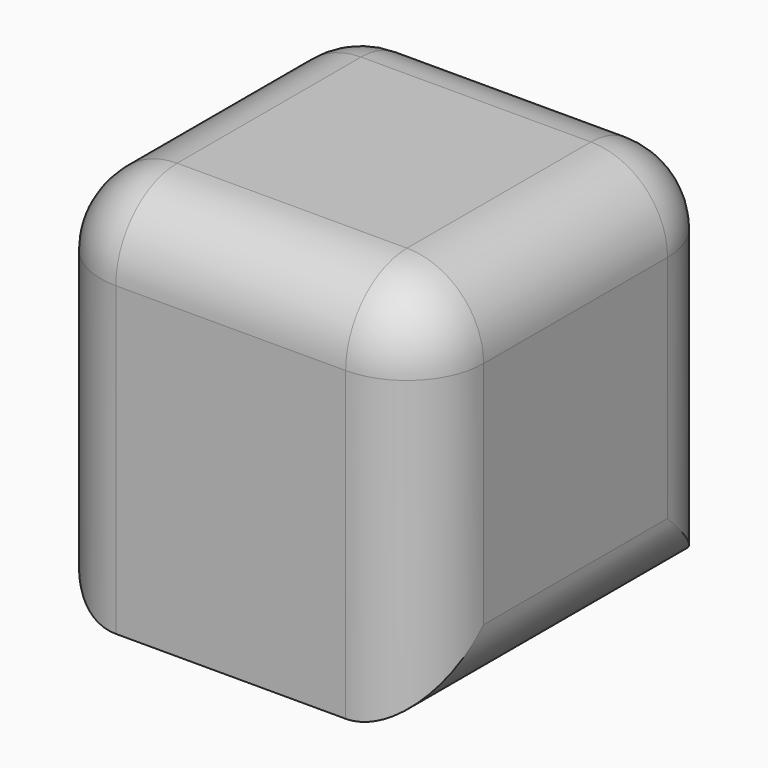
from build123d import *

# Parameters (mm, degrees)
F0_W         = 25
F0_H         = 25
F1_DEPTH     = 25
F2_T         = -3
F3_T1_DEPTH  = 32.5
F3_T3_DEPTH  = 50
F3_T5_DEPTH  = 15
F3_T7_DEPTH  = 15
F3_S11_W     = 5
F3_S11_H     = 5
F3_T12_DEPTH = 5
F3_S17_W     = 5
F3_S17_H     = 5
F3_T18_DEPTH = 5
F3_S23_W     = 5
F3_S23_H     = 5
F3_T24_DEPTH = 5
F3_S29_W     = 5
F3_S29_H     = 5
F3_T30_DEPTH = 5


# Not quite as in the source:
# - a fillet or chamfer that OpenCascade refuses, or shapes differently, is made with other operations: its cross-section is extruded or revolved along the edge and cut away or added


with BuildPart() as f1:
    # F0 (on Top) → F1 (new body)
    with BuildSketch(Plane.XY):
        with Locations((12.5, 12.5)):
            Rectangle(F0_W, F0_H)
    extrude(amount=F1_DEPTH)

    # F2
    f2_openings = [f1.faces().sort_by_distance(p)[0] for p in [
        (12.5, 12.5, 0),
    ]]
    offset(amount=F2_T, openings=f2_openings)

    # F3: fillet of radius 5 on 10 edges, made by hand

    # F3_s2 → F3_t1 (cut)
    with BuildSketch(Plane.XY.offset(-12.5)):
        with BuildLine():
            ThreePointArc((25, 20), (23.5355339059, 23.5355339059), (20, 25))
            Line((20, 25), (25, 25))
            Line((25, 25), (25, 20))
        make_face()
        with BuildLine():
            ThreePointArc((20, 0), (23.5355339059, 1.4644660941), (25, 5))
            Line((25, 5), (25, 0))
            Line((25, 0), (20, 0))
        make_face()
        with BuildLine():
            ThreePointArc((0, 20), (1.4644660941, 23.5355339059), (5, 25))
            Line((5, 25), (0, 25))
            Line((0, 25), (0, 20))
        make_face()
        with BuildLine():
            ThreePointArc((0, 5), (1.4644660941, 1.4644660941), (5, 0))
            Line((5, 0), (0, 0))
            Line((0, 0), (0, 5))
        make_face()
    extrude(amount=F3_T1_DEPTH, mode=Mode.SUBTRACT)

    # F3_s4 → F3_t3 (cut)
    with BuildSketch(Plane.XZ.offset(-37.5)):
        with BuildLine():
            ThreePointArc((25, 5), (23.5355339059, 1.4644660941), (20, 0))
            Line((20, 0), (25, 0))
            Line((25, 0), (25, 5))
        make_face()
        with BuildLine():
            ThreePointArc((0, 5), (1.4644660941, 1.4644660941), (5, 0))
            Line((5, 0), (0, 0))
            Line((0, 0), (0, 5))
        make_face()
    extrude(amount=F3_T3_DEPTH, mode=Mode.SUBTRACT)

    # F3_s6 → F3_t5 (cut)
    with BuildSketch(Plane.XZ.offset(-20)):
        with BuildLine():
            ThreePointArc((25, 20), (23.5355339059, 23.5355339059), (20, 25))
            Line((20, 25), (25, 25))
            Line((25, 25), (25, 20))
        make_face()
        with BuildLine():
            ThreePointArc((0, 20), (1.4644660941, 23.5355339059), (5, 25))
            Line((5, 25), (0, 25))
            Line((0, 25), (0, 20))
        make_face()
    extrude(amount=F3_T5_DEPTH, mode=Mode.SUBTRACT)

    # F3_s8 → F3_t7 (cut)
    with BuildSketch(Plane.YZ.offset(5)):
        with BuildLine():
            ThreePointArc((0, 20), (1.4644660941, 23.5355339059), (5, 25))
            Line((5, 25), (0, 25))
            Line((0, 25), (0, 20))
        make_face()
        with BuildLine():
            ThreePointArc((25, 20), (23.5355339059, 23.5355339059), (20, 25))
            Line((20, 25), (25, 25))
            Line((25, 25), (25, 20))
        make_face()
    extrude(amount=F3_T7_DEPTH, mode=Mode.SUBTRACT)


with BuildPart() as f3_tool10:
    # F3_s11 → F3_t12 (new body)
    with BuildSketch(Plane.YZ.offset(20)):
        with Locations((22.5, 22.5)):
            Rectangle(F3_S11_W, F3_S11_H)
    extrude(amount=F3_T12_DEPTH)

    # F3_s13 → F3_t14 (revolve, cut)
    with BuildSketch(Plane(origin=(20, 20, 20), x_dir=(0, -0.7071067812, -0.7071067812), z_dir=(0, -0.7071067812, 0.7071067812))):
        with BuildLine():
            ThreePointArc((0, -5), (5, 0), (0, 5))
            Line((0, 5), (0, -5))
        make_face()
    revolve(axis=Axis((20, 20, 20), (1, 0, 0)), mode=Mode.SUBTRACT)


with BuildPart() as f1_1:
    add(f1.part)

    # F3_t9: cut F3_tool10
    add(f3_tool10.part, mode=Mode.SUBTRACT)


with BuildPart() as f3_tool16:
    # F3_s17 → F3_t18 (new body)
    with BuildSketch(Plane.XZ.offset(-5)):
        with Locations((22.5, 22.5)):
            Rectangle(F3_S17_W, F3_S17_H)
    extrude(amount=F3_T18_DEPTH)

    # F3_s19 → F3_t20 (revolve, cut)
    with BuildSketch(Plane(origin=(20, 5, 20), x_dir=(-0.7071067812, 0, -0.7071067812), z_dir=(-0.7071067812, 0, 0.7071067812))):
        with BuildLine():
            ThreePointArc((0, -5), (5, 0), (0, 5))
            Line((0, 5), (0, -5))
        make_face()
    revolve(axis=Axis((20, 5, 20), (0, -1, 0)), mode=Mode.SUBTRACT)


with BuildPart() as f1_2:
    add(f1_1.part)

    # F3_t15: cut F3_tool16
    add(f3_tool16.part, mode=Mode.SUBTRACT)


with BuildPart() as f3_tool22:
    # F3_s23 → F3_t24 (new body)
    with BuildSketch(Plane.YZ.offset(5)):
        with Locations((22.5, 22.5)):
            Rectangle(F3_S23_W, F3_S23_H)
    extrude(amount=-F3_T24_DEPTH)

    # F3_s25 → F3_t26 (revolve, cut)
    with BuildSketch(Plane(origin=(5, 20, 20), x_dir=(0, -0.7071067812, -0.7071067812), z_dir=(0, 0.7071067812, -0.7071067812))):
        with BuildLine():
            ThreePointArc((0, -5), (5, 0), (0, 5))
            Line((0, 5), (0, -5))
        make_face()
    revolve(axis=Axis((5, 20, 20), (-1, 0, 0)), mode=Mode.SUBTRACT)


with BuildPart() as f1_3:
    add(f1_2.part)

    # F3_t21: cut F3_tool22
    add(f3_tool22.part, mode=Mode.SUBTRACT)


with BuildPart() as f3_tool28:
    # F3_s29 → F3_t30 (new body)
    with BuildSketch(Plane.YZ.offset(5)):
        with Locations((2.5, 22.5)):
            Rectangle(F3_S29_W, F3_S29_H)
    extrude(amount=-F3_T30_DEPTH)

    # F3_s31 → F3_t32 (revolve, cut)
    with BuildSketch(Plane(origin=(5, 5, 20), x_dir=(0, 0.7071067812, -0.7071067812), z_dir=(0, 0.7071067812, 0.7071067812))):
        with BuildLine():
            ThreePointArc((0, -5), (5, 0), (0, 5))
            Line((0, 5), (0, -5))
        make_face()
    revolve(axis=Axis((5, 5, 20), (-1, 0, 0)), mode=Mode.SUBTRACT)


with BuildPart() as f1_4:
    add(f1_3.part)

    # F3_t27: cut F3_tool28
    add(f3_tool28.part, mode=Mode.SUBTRACT)


solid = f1_4.part
